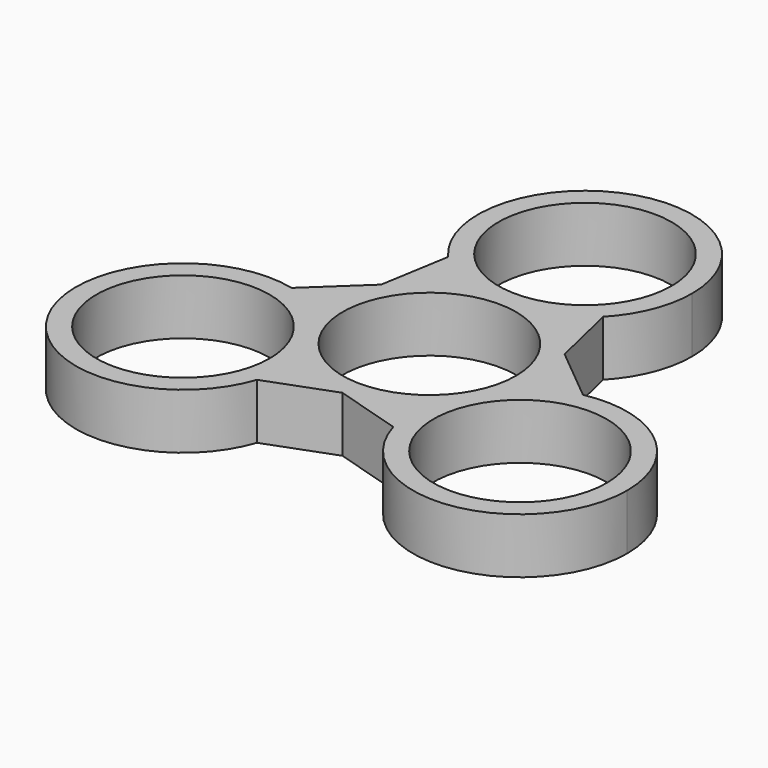
from build123d import *

# Parameters (mm, degrees)
F0_R     = 11.303
F1_DEPTH = 7.239


# Not quite as in the source:
# - a feature names something its author has since deleted; it is built from what else it names


with BuildPart() as f1:
    # F0 (on Top) → F1 (new body)
    with BuildSketch(Plane.XY):
        with BuildLine():
            ThreePointArc((-5.8198711326, 12.7), (0, 13.97), (5.8198711326, 12.7))
            ThreePointArc((5.8198711326, 12.7), (8.1011295792, 14.0187610718), (10.0941728301, 15.7424343193))
            ThreePointArc((10.0941728301, 15.7424343193), (12.9648851602, 20.1968612567), (13.97, 25.4))
            ThreePointArc((13.97, 25.4), (-4.9295356548, 38.4713648189), (-10.4910706124, 16.1751239897))
            ThreePointArc((-10.4910706124, 16.1751239897), (-8.3385146662, 14.191517803), (-5.8198711326, 12.7))
        make_face()
        with Locations((0, 25.4)):
            Circle(F0_R, mode=Mode.SUBTRACT)
        with BuildLine():
            ThreePointArc((19.2536035907, 0.9979716684), (16.4594722687, 0.1256066293), (13.9084581944, -1.3098437524))
            ThreePointArc((13.9084581944, -1.3098437524), (12.0983748909, -6.985), (8.0885870618, -11.3901562476))
            ThreePointArc((8.0885870618, -11.3901562476), (8.0900384281, -14.0251645508), (8.5862616229, -16.6130272607))
            ThreePointArc((8.5862616229, -16.6130272607), (23.9734375051, -26.5294892776), (35.9670452561, -12.7))
            ThreePointArc((35.9670452561, -12.7), (30.852411424, -1.8952144846), (19.2536035907, 0.9979716684))
        make_face()
        with Locations((21.9970452561, -12.7)):
            Circle(F0_R, mode=Mode.SUBTRACT)
        with BuildLine():
            ThreePointArc((-8.0270452561, -12.7), (-8.042439189, -12.044355651), (-8.0885870618, -11.3901562476))
            ThreePointArc((-8.0885870618, -11.3901562476), (-12.0983748909, -6.985), (-13.9084581944, -1.3098437524))
            ThreePointArc((-13.9084581944, -1.3098437524), (-16.1911680073, 0.006403479), (-18.680434453, 0.8705929414))
            ThreePointArc((-18.680434453, 0.8705929414), (-34.2395365622, -19.4292129272), (-8.7625329783, -17.1730956581))
            ThreePointArc((-8.7625329783, -17.1730956581), (-8.2121434334, -14.9665793035), (-8.0270452561, -12.7))
        make_face()
        with Locations((-21.9970452561, -12.7)):
            Circle(F0_R, mode=Mode.SUBTRACT)
        with BuildLine():
            ThreePointArc((13.9084581944, -1.3098437524), (13.9546060671, -0.655644349), (13.97, 0))
            ThreePointArc((13.97, 0), (13.5166645575, 3.5299687308), (12.1860802806, 6.8308379717))
            ThreePointArc((12.1860802806, 6.8308379717), (9.4691782802, 10.2711032853), (5.8198711326, 12.7))
            ThreePointArc((5.8198711326, 12.7), (0, 11.43), (-5.8198711326, 12.7))
            ThreePointArc((-5.8198711326, 12.7), (-9.3380147919, 10.3904946824), (-12.0087193529, 7.1380361097))
            ThreePointArc((-12.0087193529, 7.1380361097), (-13.6296255101, 3.0649973009), (-13.9084581944, -1.3098437524))
            ThreePointArc((-13.9084581944, -1.3098437524), (-9.8986703653, -5.715), (-8.0885870618, -11.3901562476))
            ThreePointArc((-8.0885870618, -11.3901562476), (-4.3294249569, -13.2822053719), (-0.1773609276, -13.9688740814))
            ThreePointArc((-0.1773609276, -13.9688740814), (4.1604472299, -13.3361005863), (8.0885870618, -11.3901562476))
            ThreePointArc((8.0885870618, -11.3901562476), (9.8986703653, -5.715), (13.9084581944, -1.3098437524))
        make_face()
        Circle(F0_R, mode=Mode.SUBTRACT)
        with BuildLine():
            ThreePointArc((-13.9084581944, -1.3098437524), (-13.6296255101, 3.0649973009), (-12.0087193529, 7.1380361097))
            Line((-12.0087193529, 7.1380361097), (-18.680434453, 0.8705929414))
            ThreePointArc((-18.680434453, 0.8705929414), (-16.1911680073, 0.006403479), (-13.9084581944, -1.3098437524))
        make_face()
        with BuildLine():
            ThreePointArc((-12.0087193529, 7.1380361097), (-9.3380147919, 10.3904946824), (-5.8198711326, 12.7))
            ThreePointArc((-5.8198711326, 12.7), (-8.3385146662, 14.191517803), (-10.4910706124, 16.1751239897))
            Line((-10.4910706124, 16.1751239897), (-12.0087193529, 7.1380361097))
        make_face()
        with BuildLine():
            ThreePointArc((5.8198711326, 12.7), (9.4691782802, 10.2711032853), (12.1860802806, 6.8308379717))
            Line((12.1860802806, 6.8308379717), (10.0941728301, 15.7424343193))
            ThreePointArc((10.0941728301, 15.7424343193), (8.1011295792, 14.0187610718), (5.8198711326, 12.7))
        make_face()
        with BuildLine():
            ThreePointArc((12.1860802806, 6.8308379717), (13.5166645575, 3.5299687308), (13.97, 0))
            ThreePointArc((13.97, 0), (13.9546060671, -0.655644349), (13.9084581944, -1.3098437524))
            ThreePointArc((13.9084581944, -1.3098437524), (16.4594722687, 0.1256066293), (19.2536035907, 0.9979716684))
            Line((19.2536035907, 0.9979716684), (12.1860802806, 6.8308379717))
        make_face()
        with BuildLine():
            ThreePointArc((8.5862616229, -16.6130272607), (8.0900384281, -14.0251645508), (8.0885870618, -11.3901562476))
            ThreePointArc((8.0885870618, -11.3901562476), (4.1604472299, -13.3361005863), (-0.1773609276, -13.9688740814))
            Line((-0.1773609276, -13.9688740814), (8.5862616229, -16.6130272607))
        make_face()
        with BuildLine():
            Line((-8.7625329783, -17.1730956581), (-0.1773609276, -13.9688740814))
            ThreePointArc((-0.1773609276, -13.9688740814), (-4.3294249569, -13.2822053719), (-8.0885870618, -11.3901562476))
            ThreePointArc((-8.0885870618, -11.3901562476), (-8.042439189, -12.044355651), (-8.0270452561, -12.7))
            ThreePointArc((-8.0270452561, -12.7), (-8.2121434334, -14.9665793035), (-8.7625329783, -17.1730956581))
        make_face()
        with BuildLine():
            ThreePointArc((8.0885870618, -11.3901562476), (12.0983748909, -6.985), (13.9084581944, -1.3098437524))
            ThreePointArc((13.9084581944, -1.3098437524), (9.8986703653, -5.715), (8.0885870618, -11.3901562476))
        make_face()
        with BuildLine():
            ThreePointArc((-5.8198711326, 12.7), (0, 11.43), (5.8198711326, 12.7))
            ThreePointArc((5.8198711326, 12.7), (0, 13.97), (-5.8198711326, 12.7))
        make_face()
        with BuildLine():
            ThreePointArc((-13.9084581944, -1.3098437524), (-12.0983748909, -6.985), (-8.0885870618, -11.3901562476))
            ThreePointArc((-8.0885870618, -11.3901562476), (-9.8986703653, -5.715), (-13.9084581944, -1.3098437524))
        make_face()
    extrude(amount=F1_DEPTH)


solid = f1.part
